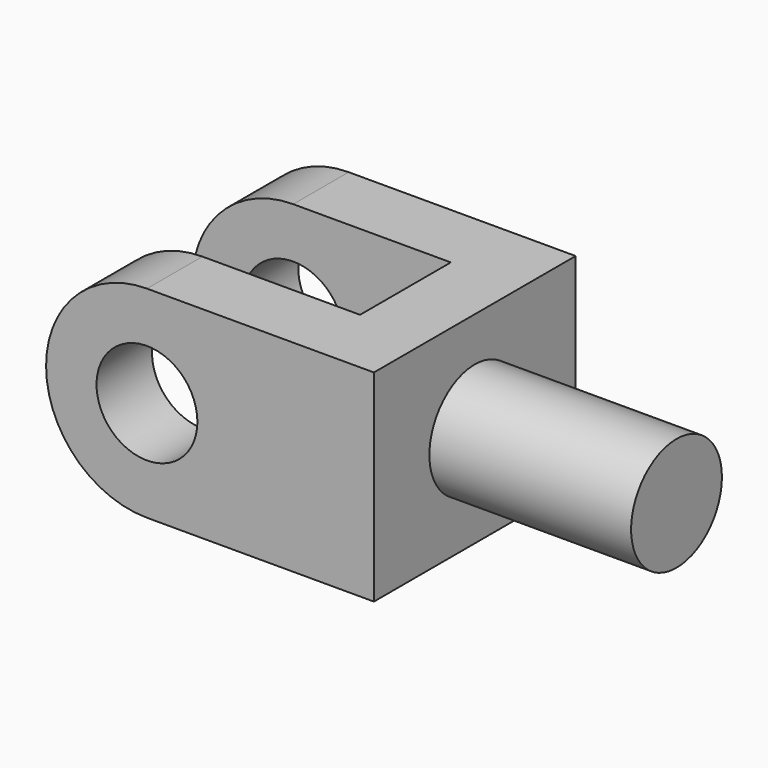
from build123d import *

# Parameters (mm, degrees)
F1_DEPTH = 81.28
F2_R     = 20.32
F3_DEPTH = 101.6
F4_R     = 40.63999
F5_R     = 40.63999
F6_R     = 22.86
F7_DEPTH = 81.28


# Not quite as in the source:
# - a fillet or chamfer is up to 0.001 mm smaller than in the source, because OpenCascade refuses the exact size


with BuildPart() as f1:
    # F0 (on Top) → F1 (new body)
    with BuildSketch(Plane.XY):
        Polygon((0, -36.7104701635), (0, 0), (0, 9.0095298365), (0, 36.9495298365), (-132.08, 36.9495298365), (-132.08, 9.0095298365), (-27.94, 9.0095298365), (-27.94, -36.7104701635), (-132.08, -36.7104701635), (-132.08, -64.6504701635), (0, -64.6504701635), align=None)
    extrude(amount=F1_DEPTH)

    # F2 (on face) → F3 (cut)
    with BuildSketch(Plane.XZ.offset(64.6504701635)):
        with Locations((-91.44, 40.64)):
            Circle(F2_R)
    extrude(amount=-F3_DEPTH, mode=Mode.SUBTRACT)

    # F4 (radius 40.64 in the source; OpenCascade refuses exactly that, so slightly less here)
    f4_edges = [f1.edges().sort_by_distance(p)[0] for p in [
        (-132.08, -50.68047, 81.28),
        (-132.08, -50.68047, 0),
    ]]
    fillet(f4_edges, radius=F4_R)

    # F5 (radius 40.64 in the source; OpenCascade refuses exactly that, so slightly less here)
    f5_edges = [f1.edges().sort_by_distance(p)[0] for p in [
        (-132.08, 22.97953, 81.28),
        (-132.08, 22.97953, 0),
    ]]
    fillet(f5_edges, radius=F5_R)

    # F6 (on face) → F7 (join)
    with BuildSketch(Plane.YZ):
        with Locations((-13.8504701635, 40.64)):
            Circle(F6_R)
    extrude(amount=F7_DEPTH)


solid = f1.part
